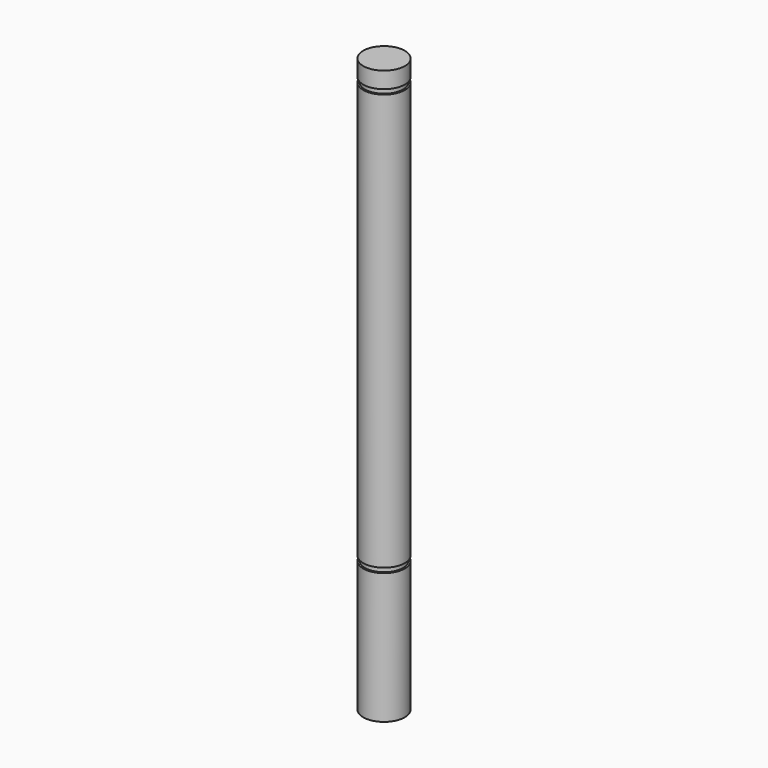
from build123d import *

# Parameters (mm, degrees)
F0_R     = 3.175
F1_DEPTH = 87.5692
F3_R     = 3.175
F3_R_2   = 2.921
F4_DEPTH = 0.7366
F6_R     = 3.175
F6_R_2   = 2.921
F7_DEPTH = 0.7366
F9_DEPTH = 6.35


# Not quite as in the source:
# - a length typed as a fraction of an inch, garbled in the dataset ("3 / 203.2 mm" for 3/8 in), is restored


with BuildPart() as f1:
    # F0 (on Top) → F1 (new body)
    with BuildSketch(Plane.XY):
        Circle(F0_R)
    extrude(amount=F1_DEPTH)

    # F3 (on offset) → F4 (cut)
    with BuildSketch(Plane(origin=(0, 0, 20), x_dir=(1, 0, 0), z_dir=(0, 0, -1))):
        Circle(F3_R)
        Circle(F3_R_2, mode=Mode.SUBTRACT)
    extrude(amount=-F4_DEPTH, mode=Mode.SUBTRACT)

    # F6 (on offset) → F7 (cut)
    with BuildSketch(Plane(origin=(0, 0, 84.3406), x_dir=(1, 0, 0), z_dir=(0, 0, -1))):
        Circle(F6_R)
        Circle(F6_R_2, mode=Mode.SUBTRACT)
    extrude(amount=-F7_DEPTH, mode=Mode.SUBTRACT)

    # F8 (on face) → F9 (cut)
    with BuildSketch(Plane(origin=(0, 0, 0), x_dir=(1, 0, 0), z_dir=(0, 0, -1))):
        with BuildLine():
            Line((2.327948453, -2.159), (-2.327948453, -2.159))
            ThreePointArc((-2.327948453, -2.159), (0, -3.175), (2.327948453, -2.159))
        make_face()
    extrude(amount=-F9_DEPTH, mode=Mode.SUBTRACT)


solid = f1.part
